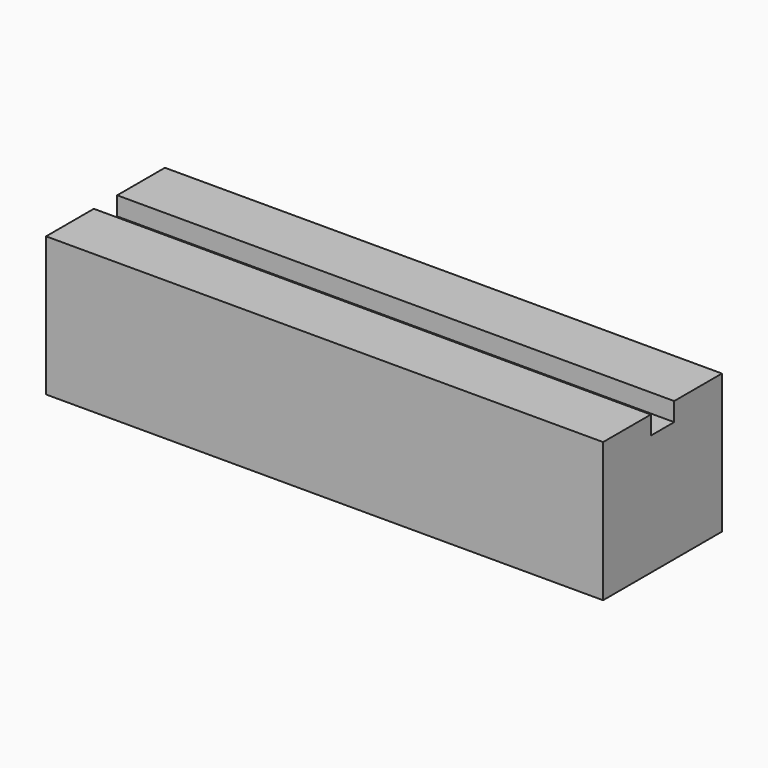
from build123d import *

# Parameters (mm, degrees)
F0_W     = 38.1
F0_H     = 10.16
F1_DEPTH = 9.525
F2_W     = 38.1
F2_H     = 1.997
F3_DEPTH = 1.27


# Not quite as in the source:
# - a length typed as a fraction of an inch, garbled in the dataset ("3 / 203.2 mm" for 3/8 in), is restored


with BuildPart() as f1:
    # F0 (on Top) → F1 (new body)
    with BuildSketch(Plane.XY):
        Rectangle(F0_W, F0_H)
    extrude(amount=-F1_DEPTH)

    # F2 (on face) → F3 (cut)
    with BuildSketch(Plane.XY):
        Rectangle(F2_W, F2_H)
    extrude(amount=-F3_DEPTH, mode=Mode.SUBTRACT)


solid = f1.part
